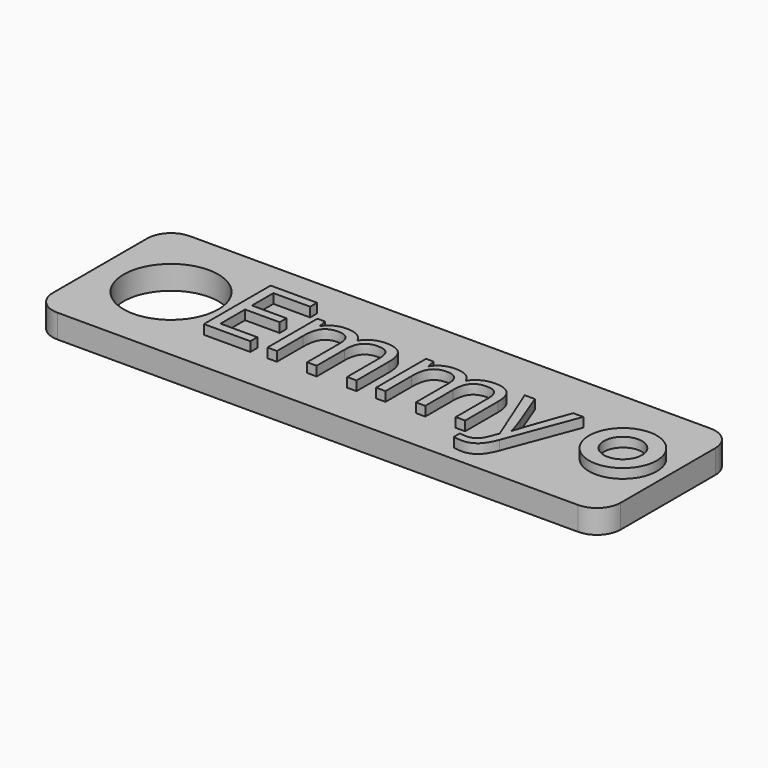
from build123d import *

# Parameters (mm, degrees)
F0_W         = 120
F0_H         = 35
F0_R         = 10
F1_DEPTH     = 5
F2_R         = 5
F3_R         = 7.1605563595
F3_R_2       = 4.0267510767
F3_TEXT_SIZE = 24.6710538502
F4_DEPTH     = 2


# Not quite as in the source:
# - Text() gives the source's letters only with a copy of the font that has no kerning and outlines rounded to 1/6400 em; it was checked with that copy


with BuildPart() as f1:
    # F0 (on Top) → F1 (new body)
    with BuildSketch(Plane.XY):
        Rectangle(F0_W, F0_H)
        with Locations((-45, 0)):
            Circle(F0_R, mode=Mode.SUBTRACT)
    extrude(amount=F1_DEPTH)

    # F2
    f2_edges = [f1.edges().sort_by_distance(p)[0] for p in [
        (-60, -17.5, 2.5),
        (60, -17.5, 2.5),
        (60, 17.5, 2.5),
        (-60, 17.5, 2.5),
    ]]
    fillet(f2_edges, radius=F2_R)

    # F3 (on face) → F4 (join)
    with BuildSketch(Plane.XY.offset(5)):
        with Locations((50.4769720137, 0)):
            Circle(F3_R)
        with Locations((50.4769720137, 0)):
            Circle(F3_R_2, mode=Mode.SUBTRACT)
        with Locations((-33.6019769311, -8.5855261423)):
            Text('Emmy', F3_TEXT_SIZE, font='Open Sans', text_align=(TextAlign.LEFT, TextAlign.BOTTOM))
    extrude(amount=F4_DEPTH)


solid = f1.part
